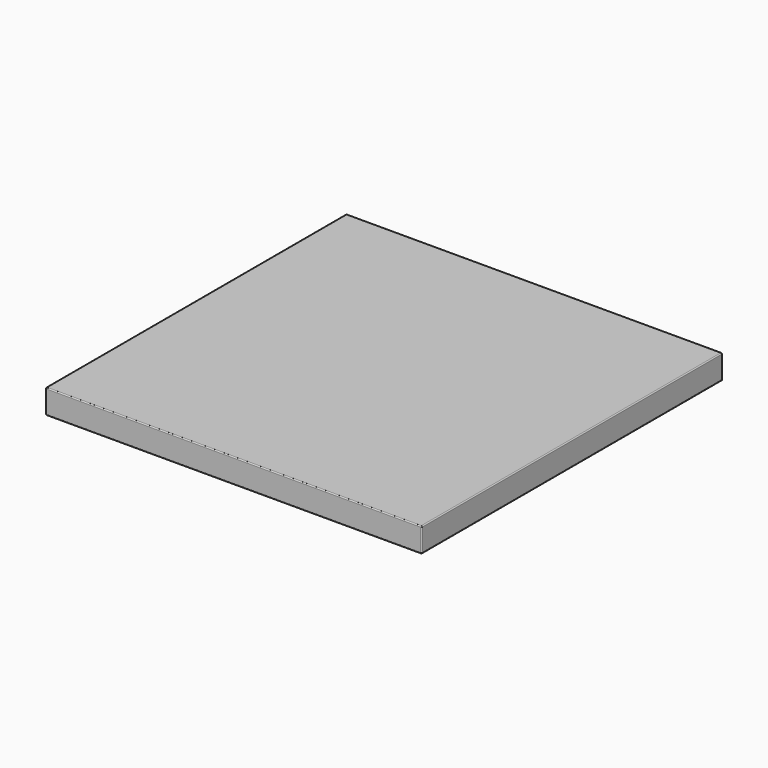
from build123d import *

# Parameters (mm, degrees)
F0_W     = 612.14
F0_H     = 612.14
F1_DEPTH = 1.5875
F3_DEPTH = 38.1
F4_R     = 1.6002
F5_R     = 1.6002
F6_R     = 1.58749
F7_R     = 1.58749


# Not quite as in the source:
# - a fillet or chamfer is up to 0.001 mm smaller than in the source, because OpenCascade refuses the exact size


with BuildPart() as f1:
    # F0 (on Top) → F1 (new body)
    with BuildSketch(Plane.XY):
        Rectangle(F0_W, F0_H)
    extrude(amount=-F1_DEPTH)

    # F2 (on face) → F3 (join)
    with BuildSketch(Plane(origin=(0, 0, -1.5875), x_dir=(1, 0, 0), z_dir=(0, 0, -1))):
        Polygon((304.4825, 304.4825), (304.4825, -306.07), (306.07, -306.07), (306.07, 306.07), (-306.07, 306.07), (-306.07, -306.07), (-304.4825, -306.07), (-304.4825, 304.4825), align=None)
    extrude(amount=F3_DEPTH)

    # F4
    f4_edges = [f1.edges().sort_by_distance(p)[0] for p in [
        (-306.07, 0, 0),
    ]]
    fillet(f4_edges, radius=F4_R)

    # F5
    f5_edges = [f1.edges().sort_by_distance(p)[0] for p in [
        (0.8001, -306.07, 0),
    ]]
    fillet(f5_edges, radius=F5_R)

    # F6 (radius 1.5875 in the source; OpenCascade refuses exactly that, so slightly less here)
    f6_edges = [f1.edges().sort_by_distance(p)[0] for p in [
        (-306.07, 0.8001, -1.6002),
        (-306.07, -304.4698, -20.64385),
        (-306.07, 306.07, -20.64385),
        (-306.07, 0.8001, -39.6875),
    ]]
    fillet(f6_edges, radius=F6_R)

    # F7 (radius 1.5875 in the source; OpenCascade refuses exactly that, so slightly less here)
    f7_edges = [f1.edges().sort_by_distance(p)[0] for p in [
        (306.07, -306.07, -19.850105),
        (306.07, -305.605035, -39.222535),
        (306.07, -305.601312, -0.468688),
        (306.07, 0.793745, -39.6875),
        (306.07, 0.006355, 0),
        (306.07, 306.07, -20.637495),
        (306.07, 305.605035, -0.464965),
    ]]
    fillet(f7_edges, radius=F7_R)


solid = f1.part
